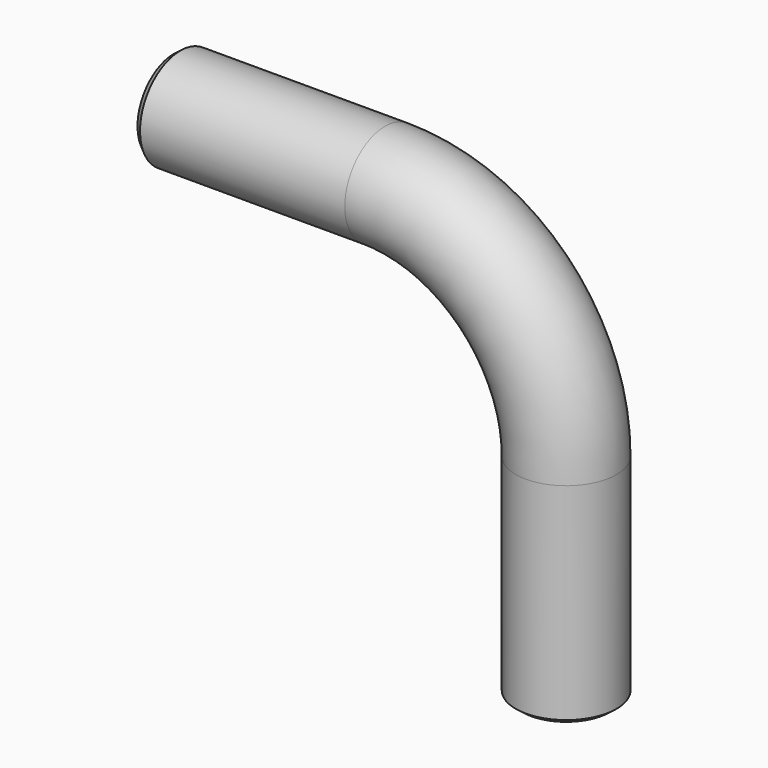
from build123d import *

# Parameters (mm, degrees)
F0_R        = 5
F0_R_2      = 4
F3_C1_SIZE2 = 0.6516126864
F3_C1_SIZE  = 0.5
F3_C2_SIZE2 = 0.5
F3_C2_SIZE  = 0.6516126864


with BuildPart() as f2:
    # F2: sweep along a path in F1
    with BuildLine(Plane.XZ) as f2_path:
        Line((0, 0), (0, 21))
        ThreePointArc((0, 21), (-5.2720779386, 33.7279220614), (-18, 39))
        Line((-18, 39), (-39, 39))
    # F0 (on Top) → F2 (sweep)
    with BuildSketch(Plane.XY):
        Circle(F0_R)
        Circle(F0_R_2, mode=Mode.SUBTRACT)
    sweep(path=f2_path.line)

    # F3: chamfer of 0.5 x 0.6516126864 on 2 edges, made by hand

    # F3_c1
    f3_c1_edges = [f2.edges().sort_by_distance(p)[0] for p in [
        (-5, 0, 0),
    ]]
    f3_c1_side = f2.faces().sort_by_distance((-5, 0, 0.01))[0]
    chamfer(f3_c1_edges, length=F3_C1_SIZE, length2=F3_C1_SIZE2, reference=f3_c1_side)

    # F3_c2
    f3_c2_edges = [f2.edges().sort_by_distance(p)[0] for p in [
        (-39, 0, 34),
    ]]
    f3_c2_side = f2.faces().sort_by_distance((-38.99, 0, 34))[0]
    chamfer(f3_c2_edges, length=F3_C2_SIZE, length2=F3_C2_SIZE2, reference=f3_c2_side)


solid = f2.part
